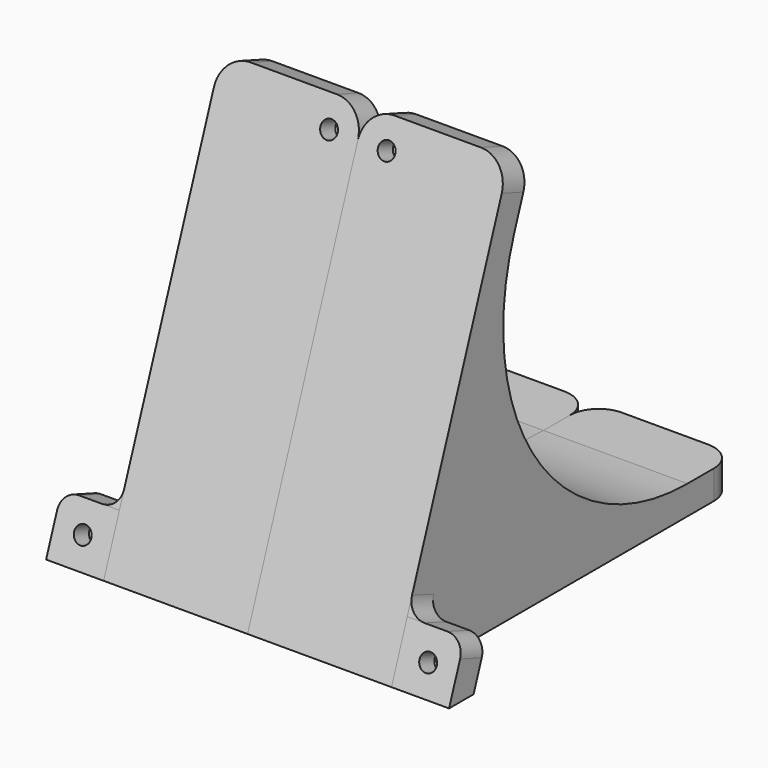
from build123d import *

# Parameters (mm, degrees)
F1_DEPTH    = 25
F3_DEPTH    = 10
F4_R        = 1.5
F5_DEPTH    = 25
F6_SIZE     = 1.5
F7_T1_DEPTH = 25
F8_R        = 5
F9_T1_DEPTH = 5
F9_T3_DEPTH = 20


# Not quite as in the source:
# - a fillet or chamfer that OpenCascade refuses, or shapes differently, is made with other operations: its cross-section is extruded or revolved along the edge and cut away or added
# - a feature names something its author has since deleted; it is built from what else it names


with BuildPart() as f1:
    # F0 (on Right) → F1 (new body)
    with BuildSketch(Plane.YZ):
        Polygon((25.6515107494, 70.4769465589), (0, 0), (75, 0), (75, 5), (7.1407400337, 5), (30.3499738534, 68.7668458423), align=None)
    extrude(amount=F1_DEPTH)

    # F2 (on face) → F3 (join)
    with BuildSketch(Plane.YZ.offset(25)):
        Polygon((8.1186645372, 7.6868254912), (3.4202014333, 9.3969262079), (0, 0), (5.3208888624, 0), (7.1407400337, 5), align=None)
    extrude(amount=F3_DEPTH)

    # F4 (on face) → F5 (cut)
    with BuildSketch(Plane(origin=(0, 0, 0), x_dir=(1, 0, 0), z_dir=(0, -0.9396926208, 0.3420201433))):
        with Locations((30, 5)):
            Circle(F4_R)
        with Locations((5, 70)):
            Circle(F4_R)
    extrude(amount=-F5_DEPTH, mode=Mode.SUBTRACT)

    # F6
    f6_edges = [f1.edges().sort_by_distance(p)[0] for p in [
        (28.5, 6.408564, 2.988362),
        (3.5, 28.639873, 64.068383),
    ]]
    chamfer(f6_edges, length=F6_SIZE)

    # F7: fillet of radius 40 on 1 edges, made by hand

    # F7_s2 → F7_t1 (join)
    with BuildSketch(Plane.YZ):
        with BuildLine():
            ThreePointArc((26.678955472, 58.680805733), (31.5005785318, 22.056942546), (64.2666603034, 5))
            Line((64.2666603034, 5), (7.1407400337, 5))
            Line((7.1407400337, 5), (26.678955472, 58.680805733))
        make_face()
    extrude(amount=F7_T1_DEPTH)

    # F8
    f8_edges = [f1.edges().sort_by_distance(p)[0] for p in [
        (25, 28.000742, 69.621896),
        (0, 28.000742, 69.621896),
        (0, 75, 2.5),
        (25, 75, 2.5),
    ]]
    fillet(f8_edges, radius=F8_R)

    # F9: fillet of radius 3 on 2 edges, made by hand

    # F9_s2 → F9_t1 (join)
    with BuildSketch(Plane(origin=(0, 4.6984631039, -1.7101007166), x_dir=(1, 0, 0), z_dir=(0, -0.9396926208, 0.3420201433))):
        with BuildLine():
            ThreePointArc((25, 13), (25.8786796564, 10.8786796564), (28, 10))
            Line((28, 10), (25, 10))
            Line((25, 10), (25, 13))
        make_face()
    extrude(amount=F9_T1_DEPTH)

    # F9_s4 → F9_t3 (cut)
    with BuildSketch(Plane(origin=(0, 11.7461577598, -4.2752517916), x_dir=(1, 0, 0), z_dir=(0, -0.9396926208, 0.3420201433))):
        with BuildLine():
            ThreePointArc((35, 7), (34.1213203436, 9.1213203436), (32, 10))
            Line((32, 10), (35, 10))
            Line((35, 10), (35, 7))
        make_face()
    extrude(amount=F9_T3_DEPTH, mode=Mode.SUBTRACT)


with BuildPart() as f10_1:
    # F10: instance of F1
    add(f1.part.mirror(Plane.YZ))


solid = Compound([f1.part, f10_1.part])
